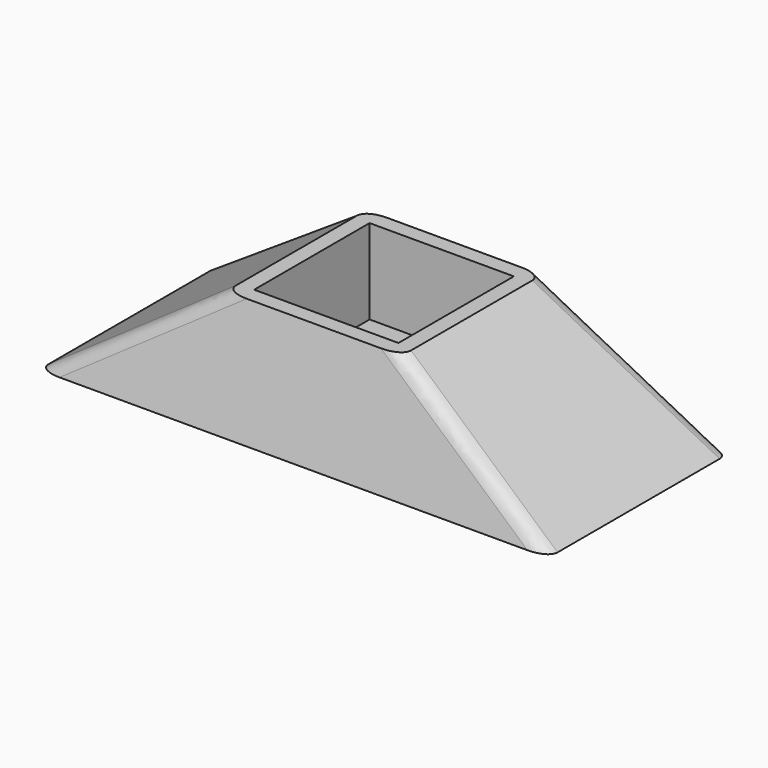
from build123d import *

# Parameters (mm, degrees)
F0_W        = 180
F0_H        = 80
F2_W        = 62
F2_H        = 62
F4_W        = 51
F4_H        = 51
F5_DEPTH    = 30
F6_T        = 5
F6_T3_DEPTH = 40
F6_T5_DEPTH = 61
F6_T7_DEPTH = 61
F7_R        = 5


# Not quite as in the source:
# - a shell that OpenCascade refuses in one call is made with other operations: the cavity is built on its own and cut out


with BuildPart() as f3:
    # F0 (on Top) → F3 section 0
    with BuildSketch(Plane.XY):
        Rectangle(F0_W, F0_H)
    # F2 (on offset) → F3 section 1
    with BuildSketch(Plane.XY.offset(40)):
        Rectangle(F2_W, F2_H)
    loft()

    # F4 (on face) → F5 (cut)
    with BuildSketch(Plane.XY.offset(40)):
        Rectangle(F4_W, F4_H)
    extrude(amount=-F5_DEPTH, mode=Mode.SUBTRACT)

    # F6: shell of thickness 5, made by hand


with BuildPart() as f6_core1:
    # F6_t2: copy of F3
    add(f3.part)

    # the walls: a layer under each face that stays
    f6_faces = [f6_core1.faces().sort_by_distance(p)[0] for p in [
        (0, 35.5, 20),
        (-60.5, 0, 20),
        (26.5714285714, 26.5714285714, 40),
        (60.5, 0, 20),
        (0, -35.5, 20),
        (-25.5, 0, 25),
        (0, 25.5, 25),
        (25.5, 0, 25),
        (0, -25.5, 25),
        (0, 0, 10),
    ]]
    thicken(f6_faces, amount=-F6_T, mode=Mode.SUBTRACT)

    # F6_s4 → F6_t3 (cut)
    with BuildSketch(Plane.XY.offset(5)):
        Polygon((-25.45, 25.45), (-30.5, 25.5), (-30.5, 30.5), (-25.5, 30.5), align=None)
        Polygon((-25.45, -25.45), (-30.5, -25.5), (-30.5, -30.5), (-25.5, -30.5), align=None)
        Polygon((25.45, 25.45), (25.5, 30.5), (30.5, 30.5), (30.5, 25.5), align=None)
        Polygon((25.45, -25.45), (30.5, -25.5), (30.5, -30.5), (25.5, -30.5), align=None)
    extrude(amount=F6_T3_DEPTH, mode=Mode.SUBTRACT)

    # F6_s6 → F6_t5 (cut)
    with BuildSketch(Plane.XZ.offset(-30.5)):
        Polygon((-25.45, 10.05), (-30.5, 10), (-30.5, 5), (-25.5, 5), align=None)
        Polygon((25.45, 10.05), (30.5, 10), (30.5, 5), (25.5, 5), align=None)
    extrude(amount=F6_T5_DEPTH, mode=Mode.SUBTRACT)

    # F6_s8 → F6_t7 (cut)
    with BuildSketch(Plane.YZ.offset(-30.5)):
        Polygon((25.45, 10.05), (30.5, 10), (30.5, 5), (25.5, 5), align=None)
        Polygon((-25.45, 10.05), (-30.5, 10), (-30.5, 5), (-25.5, 5), align=None)
    extrude(amount=F6_T7_DEPTH, mode=Mode.SUBTRACT)


with BuildPart() as f3_1:
    add(f3.part)

    # what is left inside the walls is the cavity
    f6_cavity = [f6_core1.part.solids().sort_by_distance(p)[0] for p in [
        (8.772982, -19.739209, 0.05),
    ]]
    add(f6_cavity, mode=Mode.SUBTRACT)

    # F7
    f7_edges = [f3_1.edges().sort_by_distance(p)[0] for p in [
        (60.5, -35.5, 20),
        (60.5, 35.5, 20),
        (-60.5, 35.5, 20),
        (-60.5, -35.5, 20),
    ]]
    fillet(f7_edges, radius=F7_R)


solid = f3_1.part
